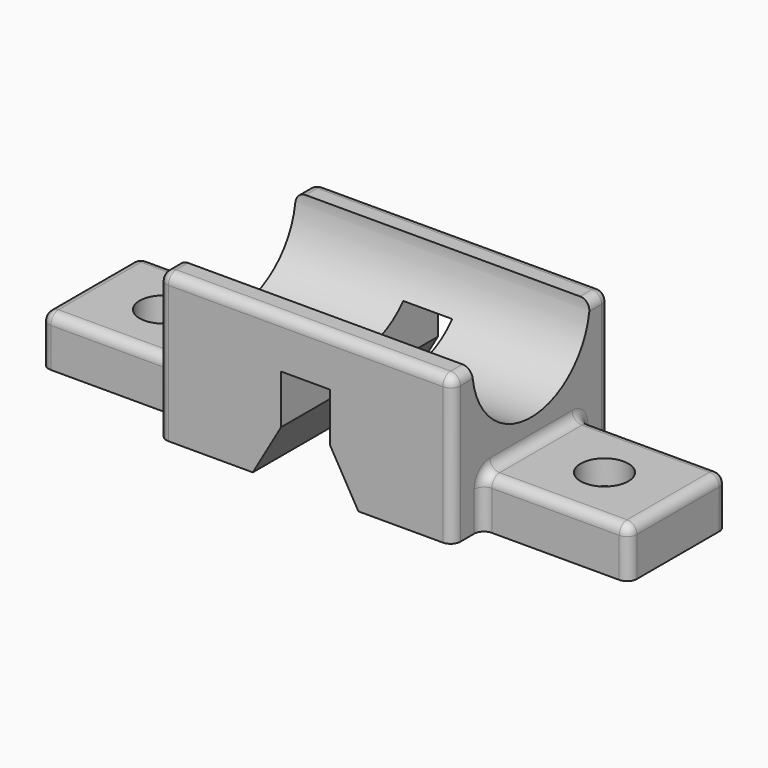
from build123d import *

# Parameters (mm, degrees)
F0_W           = 60
F0_H           = 40
F1_DEPTH       = 30
F3_DEPTH       = 40.001
F4_R           = 15
F5_DEPTH       = 40
F6_W           = 25
F6_H           = 10
F7_DEPTH       = 30
F9_D           = 5.5
F9_CBORE_D     = 9.75
F9_CBORE_DEPTH = 5
F10_T1_DEPTH   = 13
F10_T3_DEPTH   = 28
F10_T5_DEPTH   = 21
F10_T7_DEPTH   = 33
F10_T9_DEPTH   = 8
F10_T11_DEPTH  = 56
F10_T13_DEPTH  = 8
F10_S17_W      = 2
F10_S17_H      = 2
F10_T18_DEPTH  = 2
F10_S23_W      = 2
F10_S23_H      = 2
F10_T24_DEPTH  = 2
F10_S29_W      = 2
F10_S29_H      = 2
F10_T30_DEPTH  = 2
F10_S35_W      = 2
F10_S35_H      = 2
F10_T36_DEPTH  = 2
F10_S41_W      = 2
F10_S41_H      = 2
F10_T42_DEPTH  = 2
F10_S47_W      = 2
F10_S47_H      = 2
F10_T48_DEPTH  = 2
F10_T51_DEPTH  = 8
F10_T53_DEPTH  = 21
F10_T56_ANGLE  = 90
F10_T58_ANGLE  = 90


# Not quite as in the source:
# - a fillet or chamfer that OpenCascade refuses, or shapes differently, is made with other operations: its cross-section is extruded or revolved along the edge and cut away or added


with BuildPart() as f1:
    # F0 (on Top) → F1 (new body)
    with BuildSketch(Plane.XY):
        Rectangle(F0_W, F0_H)
    extrude(amount=F1_DEPTH)

    # F2 (on face) → F3 (cut, through all)
    with BuildSketch(Plane.XZ.offset(20)):
        Polygon((-5, 10), (-10.7735026919, 0), (10.7735026919, 0), (5, 10), (5, 20), (-5, 20), align=None)
    extrude(amount=-F3_DEPTH, mode=Mode.SUBTRACT)

    # F4 (on Right) → F5 (cut, symmetric)
    with BuildSketch(Plane.YZ):
        with Locations((0, 30)):
            Circle(F4_R)
    extrude(amount=F5_DEPTH, both=True, mode=Mode.SUBTRACT)

    # F6 (on face) → F7 (join)
    with BuildSketch(Plane.YZ.offset(30)):
        with Locations((0, 5)):
            Rectangle(F6_W, F6_H)
    extrude(amount=F7_DEPTH)

    # F9 (through all)
    with Locations(Plane.XY.offset(10)):
        with Locations((45, 0)):
            CounterBoreHole(F9_D / 2, F9_CBORE_D / 2, F9_CBORE_DEPTH)

    # F10: fillet of radius 2 on 18 edges, made by hand

    # F10_s2 → F10_t1 (cut)
    with BuildSketch(Plane.XY.offset(-5)):
        with BuildLine():
            ThreePointArc((58, -12.5), (59.4142135624, -11.9142135624), (60, -10.5))
            Line((60, -10.5), (60, -12.5))
            Line((60, -12.5), (58, -12.5))
        make_face()
        with BuildLine():
            ThreePointArc((60, 10.5), (59.4142135624, 11.9142135624), (58, 12.5))
            Line((58, 12.5), (60, 12.5))
            Line((60, 12.5), (60, 10.5))
        make_face()
    extrude(amount=F10_T1_DEPTH, mode=Mode.SUBTRACT)

    # F10_s4 → F10_t3 (cut)
    with BuildSketch(Plane.YZ.offset(30)):
        with BuildLine():
            ThreePointArc((-12.5, 8), (-11.9142135624, 9.4142135624), (-10.5, 10))
            Line((-10.5, 10), (-12.5, 10))
            Line((-12.5, 10), (-12.5, 8))
        make_face()
        with BuildLine():
            ThreePointArc((12.5, 8), (11.9142135624, 9.4142135624), (10.5, 10))
            Line((10.5, 10), (12.5, 10))
            Line((12.5, 10), (12.5, 8))
        make_face()
    extrude(amount=F10_T3_DEPTH, mode=Mode.SUBTRACT)

    # F10_s6 → F10_t5 (cut)
    with BuildSketch(Plane.XZ.offset(-10.5)):
        with BuildLine():
            ThreePointArc((60, 8), (59.4142135624, 9.4142135624), (58, 10))
            Line((58, 10), (60, 10))
            Line((60, 10), (60, 8))
        make_face()
    extrude(amount=F10_T5_DEPTH, mode=Mode.SUBTRACT)

    # F10_s8 → F10_t7 (cut)
    with BuildSketch(Plane.XY.offset(-5)):
        with BuildLine():
            ThreePointArc((30, -18), (29.4142135624, -19.4142135624), (28, -20))
            Line((28, -20), (30, -20))
            Line((30, -20), (30, -18))
        make_face()
        with BuildLine():
            ThreePointArc((28, 20), (29.4142135624, 19.4142135624), (30, 18))
            Line((30, 18), (30, 20))
            Line((30, 20), (28, 20))
        make_face()
        with BuildLine():
            ThreePointArc((-30, -18), (-29.4142135624, -19.4142135624), (-28, -20))
            Line((-28, -20), (-30, -20))
            Line((-30, -20), (-30, -18))
        make_face()
        with BuildLine():
            ThreePointArc((-28, 20), (-29.4142135624, 19.4142135624), (-30, 18))
            Line((-30, 18), (-30, 20))
            Line((-30, 20), (-28, 20))
        make_face()
    extrude(amount=F10_T7_DEPTH, mode=Mode.SUBTRACT)

    # F10_s10 → F10_t9 (cut)
    with BuildSketch(Plane.XZ.offset(10)):
        with BuildLine():
            ThreePointArc((30, 28), (29.4142135624, 29.4142135624), (28, 30))
            Line((28, 30), (30, 30))
            Line((30, 30), (30, 28))
        make_face()
        with BuildLine():
            ThreePointArc((-30, 28), (-29.4142135624, 29.4142135624), (-28, 30))
            Line((-28, 30), (-30, 30))
            Line((-30, 30), (-30, 28))
        make_face()
    extrude(amount=F10_T9_DEPTH, mode=Mode.SUBTRACT)

    # F10_s12 → F10_t11 (cut)
    with BuildSketch(Plane.YZ.offset(-28)):
        with BuildLine():
            ThreePointArc((20, 28), (19.4142135624, 29.4142135624), (18, 30))
            Line((18, 30), (20, 30))
            Line((20, 30), (20, 28))
        make_face()
        with BuildLine():
            ThreePointArc((-20, 28), (-19.4142135624, 29.4142135624), (-18, 30))
            Line((-18, 30), (-20, 30))
            Line((-20, 30), (-20, 28))
        make_face()
    extrude(amount=F10_T11_DEPTH, mode=Mode.SUBTRACT)

    # F10_s14 → F10_t13 (cut)
    with BuildSketch(Plane.XZ.offset(-18)):
        with BuildLine():
            ThreePointArc((-30, 28), (-29.4142135624, 29.4142135624), (-28, 30))
            Line((-28, 30), (-30, 30))
            Line((-30, 30), (-30, 28))
        make_face()
        with BuildLine():
            ThreePointArc((28, 30), (29.4142135624, 29.4142135624), (30, 28))
            Line((30, 28), (30, 30))
            Line((30, 30), (28, 30))
        make_face()
    extrude(amount=F10_T13_DEPTH, mode=Mode.SUBTRACT)


with BuildPart() as f10_tool16:
    # F10_s17 → F10_t18 (new body)
    with BuildSketch(Plane.XY.offset(8)):
        with Locations((59, -11.5)):
            Rectangle(F10_S17_W, F10_S17_H)
    extrude(amount=F10_T18_DEPTH)

    # F10_s19 → F10_t20 (revolve, cut)
    with BuildSketch(Plane(origin=(58, -10.5, 8), x_dir=(-0.7071067812, 0.7071067812, 0), z_dir=(0.7071067812, 0.7071067812, 0))):
        with BuildLine():
            ThreePointArc((0, -2), (2, 0), (0, 2))
            Line((0, 2), (0, -2))
        make_face()
    revolve(axis=Axis((58, -10.5, 8), (0, 0, 1)), mode=Mode.SUBTRACT)


with BuildPart() as f1_1:
    add(f1.part)

    # F10_t15: cut F10_tool16
    add(f10_tool16.part, mode=Mode.SUBTRACT)


with BuildPart() as f10_tool22:
    # F10_s23 → F10_t24 (new body)
    with BuildSketch(Plane.XY.offset(8)):
        with Locations((59, 11.5)):
            Rectangle(F10_S23_W, F10_S23_H)
    extrude(amount=F10_T24_DEPTH)

    # F10_s25 → F10_t26 (revolve, cut)
    with BuildSketch(Plane(origin=(58, 10.5, 8), x_dir=(-0.7071067812, -0.7071067812, 0), z_dir=(-0.7071067812, 0.7071067812, 0))):
        with BuildLine():
            ThreePointArc((0, -2), (2, 0), (0, 2))
            Line((0, 2), (0, -2))
        make_face()
    revolve(axis=Axis((58, 10.5, 8), (0, 0, 1)), mode=Mode.SUBTRACT)


with BuildPart() as f1_2:
    add(f1_1.part)

    # F10_t21: cut F10_tool22
    add(f10_tool22.part, mode=Mode.SUBTRACT)


with BuildPart() as f10_tool28:
    # F10_s29 → F10_t30 (new body)
    with BuildSketch(Plane.XY.offset(28)):
        with Locations((29, -19)):
            Rectangle(F10_S29_W, F10_S29_H)
    extrude(amount=F10_T30_DEPTH)

    # F10_s31 → F10_t32 (revolve, cut)
    with BuildSketch(Plane(origin=(28, -18, 28), x_dir=(-0.7071067812, 0.7071067812, 0), z_dir=(0.7071067812, 0.7071067812, 0))):
        with BuildLine():
            ThreePointArc((0, -2), (2, 0), (0, 2))
            Line((0, 2), (0, -2))
        make_face()
    revolve(axis=Axis((28, -18, 28), (0, 0, 1)), mode=Mode.SUBTRACT)


with BuildPart() as f1_3:
    add(f1_2.part)

    # F10_t27: cut F10_tool28
    add(f10_tool28.part, mode=Mode.SUBTRACT)


with BuildPart() as f10_tool34:
    # F10_s35 → F10_t36 (new body)
    with BuildSketch(Plane.YZ.offset(-28)):
        with Locations((-19, 29)):
            Rectangle(F10_S35_W, F10_S35_H)
    extrude(amount=-F10_T36_DEPTH)

    # F10_s37 → F10_t38 (revolve, cut)
    with BuildSketch(Plane(origin=(-28, -18, 28), x_dir=(0, 0.7071067812, -0.7071067812), z_dir=(0, 0.7071067812, 0.7071067812))):
        with BuildLine():
            ThreePointArc((0, -2), (2, 0), (0, 2))
            Line((0, 2), (0, -2))
        make_face()
    revolve(axis=Axis((-28, -18, 28), (-1, 0, 0)), mode=Mode.SUBTRACT)


with BuildPart() as f1_4:
    add(f1_3.part)

    # F10_t33: cut F10_tool34
    add(f10_tool34.part, mode=Mode.SUBTRACT)


with BuildPart() as f10_tool40:
    # F10_s41 → F10_t42 (new body)
    with BuildSketch(Plane.XZ.offset(-18)):
        with Locations((29, 29)):
            Rectangle(F10_S41_W, F10_S41_H)
    extrude(amount=-F10_T42_DEPTH)

    # F10_s43 → F10_t44 (revolve, cut)
    with BuildSketch(Plane(origin=(28, 18, 28), x_dir=(-0.7071067812, 0, -0.7071067812), z_dir=(0.7071067812, 0, -0.7071067812))):
        with BuildLine():
            ThreePointArc((0, -2), (2, 0), (0, 2))
            Line((0, 2), (0, -2))
        make_face()
    revolve(axis=Axis((28, 18, 28), (0, 1, 0)), mode=Mode.SUBTRACT)


with BuildPart() as f1_5:
    add(f1_4.part)

    # F10_t39: cut F10_tool40
    add(f10_tool40.part, mode=Mode.SUBTRACT)


with BuildPart() as f10_tool46:
    # F10_s47 → F10_t48 (new body)
    with BuildSketch(Plane.XZ.offset(-18)):
        with Locations((-29, 29)):
            Rectangle(F10_S47_W, F10_S47_H)
    extrude(amount=-F10_T48_DEPTH)

    # F10_s49 → F10_t50 (revolve, cut)
    with BuildSketch(Plane(origin=(-28, 18, 28), x_dir=(0.7071067812, 0, -0.7071067812), z_dir=(0.7071067812, 0, 0.7071067812))):
        with BuildLine():
            ThreePointArc((0, -2), (2, 0), (0, 2))
            Line((0, 2), (0, -2))
        make_face()
    revolve(axis=Axis((-28, 18, 28), (0, 1, 0)), mode=Mode.SUBTRACT)


with BuildPart() as f1_6:
    add(f1_5.part)

    # F10_t45: cut F10_tool46
    add(f10_tool46.part, mode=Mode.SUBTRACT)

    # F10_s52 → F10_t51 (join)
    with BuildSketch(Plane.XY):
        with BuildLine():
            ThreePointArc((30, -14.5), (30.5857864376, -13.0857864376), (32, -12.5))
            Line((32, -12.5), (30, -12.5))
            Line((30, -12.5), (30, -14.5))
        make_face()
        with BuildLine():
            ThreePointArc((30, 14.5), (30.5857864376, 13.0857864376), (32, 12.5))
            Line((32, 12.5), (30, 12.5))
            Line((30, 12.5), (30, 14.5))
        make_face()
    extrude(amount=F10_T51_DEPTH)

    # F10_s54 → F10_t53 (join)
    with BuildSketch(Plane.XZ.offset(-10.5)):
        with BuildLine():
            ThreePointArc((30, 12), (30.5857864376, 10.5857864376), (32, 10))
            Line((32, 10), (30, 10))
            Line((30, 10), (30, 12))
        make_face()
    extrude(amount=F10_T53_DEPTH)

    # F10_s55 → F10_t56 (revolve)
    with BuildSketch(Plane.XY.offset(8)):
        with BuildLine():
            ThreePointArc((30, 14.5), (30.5857864376, 13.0857864376), (32, 12.5))
            Line((32, 12.5), (30, 12.5))
            Line((30, 12.5), (30, 14.5))
        make_face()
    revolve(axis=Axis((30, 10.5, 8), (1, 0, 0)), revolution_arc=F10_T56_ANGLE)

    # F10_s57 → F10_t58 (revolve)
    with BuildSketch(Plane.XY.offset(8)):
        with BuildLine():
            ThreePointArc((30, -14.5), (30.5857864376, -13.0857864376), (32, -12.5))
            Line((32, -12.5), (30, -12.5))
            Line((30, -12.5), (30, -14.5))
        make_face()
    revolve(axis=Axis((30, -10.5, 8), (-1, 0, 0)), revolution_arc=F10_T58_ANGLE)

    # F11: F1 across plane


with BuildPart() as f1_7:
    add(f1_6.part)
    add(f1_6.part.mirror(Plane.YZ))


solid = f1_7.part
